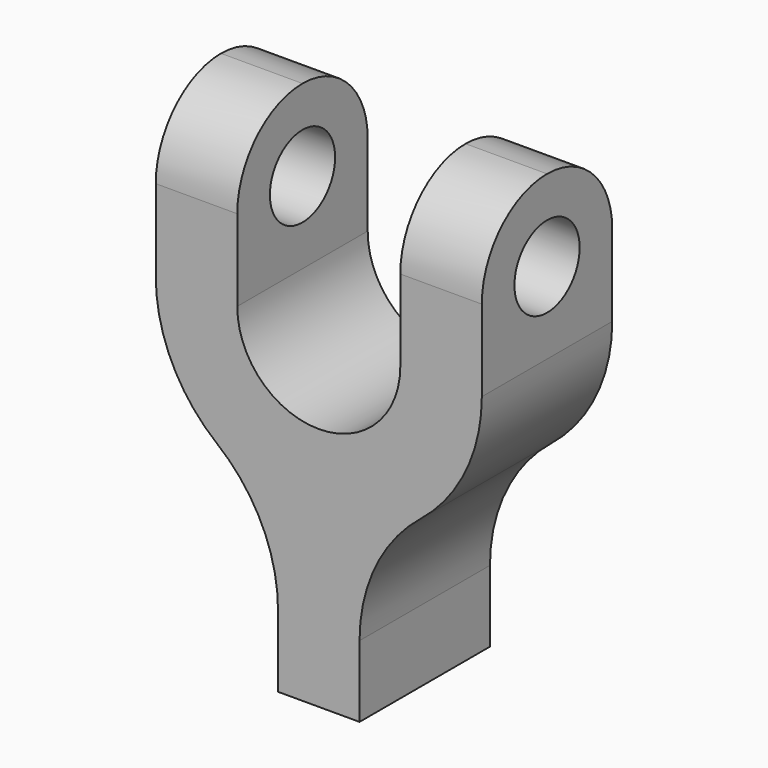
from build123d import *

# Parameters (mm, degrees)
F1_DEPTH      = 5
F2_R          = 4.99999
F3_R          = 2.5
F4_DEPTH      = 10.001
F4_DEPTH_BACK = 10.001


# Not quite as in the source:
# - a fillet or chamfer is up to 0.001 mm smaller than in the source, because OpenCascade refuses the exact size


with BuildPart() as f1:
    # F0 (on Front) → F1 (new body, symmetric)
    with BuildSketch(Plane.XZ):
        with BuildLine():
            Line((0, -15), (2.5, -15))
            Line((2.5, -15), (2.5, -10.612494996))
            ThreePointArc((2.5, -10.612494996), (3.4861218113, -6.2823679771), (6.25, -2.806247498))
            ThreePointArc((6.25, -2.806247498), (9.0138781887, 0.6698729811), (10, 5))
            Line((10, 5), (10, 15))
            Line((10, 15), (5, 15))
            Line((5, 15), (5, 5))
            ThreePointArc((5, 5), (3.5355339059, 1.4644660941), (0, 0))
            ThreePointArc((0, 0), (-3.5355339059, 1.4644660941), (-5, 5))
            Line((-5, 5), (-5, 15))
            Line((-5, 15), (-10, 15))
            Line((-10, 15), (-10, 5))
            ThreePointArc((-10, 5), (-9.0138781887, 0.6698729811), (-6.25, -2.806247498))
            ThreePointArc((-6.25, -2.806247498), (-3.4861218113, -6.2823679771), (-2.5, -10.612494996))
            Line((-2.5, -10.612494996), (-2.5, -15))
            Line((-2.5, -15), (0, -15))
        make_face()
    extrude(amount=F1_DEPTH, both=True)

    # F2 (radius 5 in the source; OpenCascade refuses exactly that, so slightly less here)
    f2_edges = [f1.edges().sort_by_distance(p)[0] for p in [
        (-7.5, -5, 15),
        (7.5, -5, 15),
        (7.5, 5, 15),
        (-7.5, 5, 15),
    ]]
    fillet(f2_edges, radius=F2_R)

    # F3 (on Right) → F4 (cut, two sides)
    with BuildSketch(Plane.YZ) as f4_sk:
        with Locations((0, 10)):
            Circle(F3_R)
    extrude(amount=-F4_DEPTH, mode=Mode.SUBTRACT)
    extrude(f4_sk.sketch, amount=F4_DEPTH_BACK, mode=Mode.SUBTRACT)


solid = f1.part
